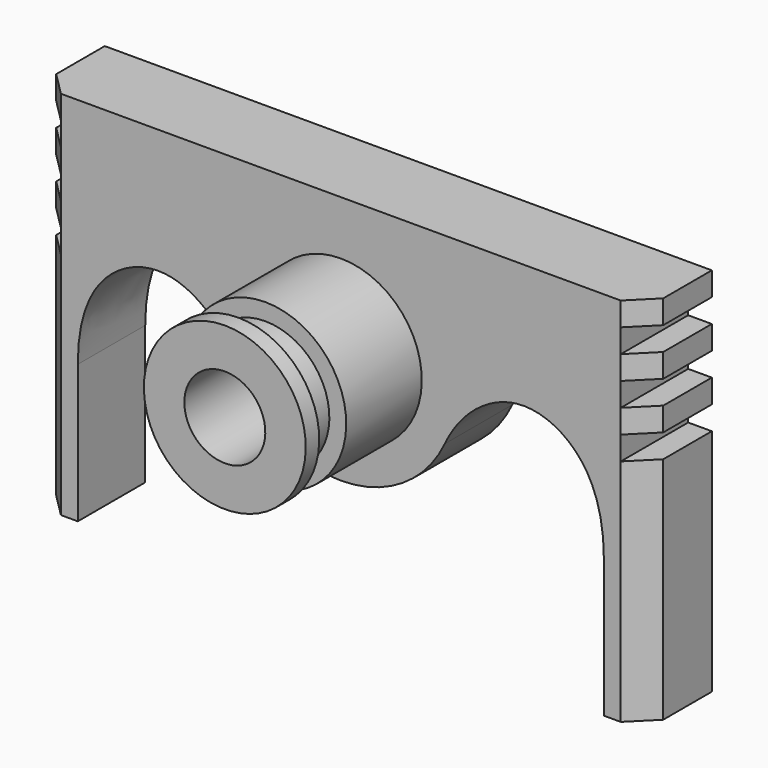
from build123d import *
from build123d import SkipClean  # not in build123d's __all__

# Parameters (mm, degrees)
F1_DEPTH = 2.5
F4_SIZE  = 0.7
F3_W     = 2.5
F3_H     = 1.2


with BuildPart() as f1:
    # F0 (on Front) → F1 (new body)
    with BuildSketch(Plane.XZ):
        with BuildLine():
            Line((0, 4), (-9, 4))
            Line((-9, 4), (-9, 3.3))
            Line((-9, 3.3), (-8.3, 3.3))
            Line((-8.3, 3.3), (-8.3, 2.6))
            Line((-8.3, 2.6), (-9, 2.6))
            Line((-9, 2.6), (-9, 1.9))
            Line((-9, 1.9), (-8.3, 1.9))
            Line((-8.3, 1.9), (-8.3, 1.2))
            Line((-8.3, 1.2), (-9, 1.2))
            Line((-9, 1.2), (-9, 0.5))
            Line((-9, 0.5), (-8.3, 0.5))
            Line((-8.3, 0.5), (-8.3, -0.2))
            Line((-8.3, -0.2), (-9, -0.2))
            Line((-9, -0.2), (-9, -7))
            Line((-9, -7), (-7.8, -7))
            Line((-7.8, -7), (-7.8, -2.900873477))
            add(Edge.make_bspline(
                [(-7.8, -2.900873477), (-7.8, -1.685574969), (-7.1826716424, -0.1281665724), (-4.9759016066, 0.6847768295), (-3.5267368498, -0.4819738014), (-3.0814464759, -1.4369020899)],
                knots=[0, 0, 0, 0, 0.3572792207, 0.6508868549, 1, 1, 1, 1], degree=3))
            ThreePointArc((-3.0814464759, -1.4369020899), (-1.8268186684, -2.8675309158), (0, -3.4))
            Line((0, -3.4), (0, -2.4))
            ThreePointArc((0, -2.4), (-2.4, 0), (0, 2.4))
            Line((0, 2.4), (0, 4))
        make_face()
    extrude(amount=F1_DEPTH)

    # F2: F1 across plane


with BuildPart() as f1_1:
    add(f1.part, clean=False)
    with SkipClean():  # cleaning this boolean's faces spoils the solid; the shape is the same uncleaned
        add(f1.part.mirror(Plane.YZ), clean=False)

    # F4
    f4_edges = [f1_1.edges().sort_by_distance(p)[0] for p in [
        (-9, -2.5, -3.6),
        (9, -2.5, -3.6),
        (-9, -2.5, 3.65),
        (-9, -2.5, 2.25),
        (-9, -2.5, 0.85),
        (9, -2.5, 3.65),
        (9, -2.5, 2.25),
        (9, -2.5, 0.85),
    ]]
    chamfer(f4_edges, length=F4_SIZE)

    # F3 (on Right) → F5 (revolve)
    with BuildSketch(Plane.YZ):
        Polygon((-2.5, 1.2), (-2.5, 2.4), (-5.3, 2.4), (-5.3, 1.9), (-6.3, 1.9), (-6.3, 2.4), (-6.8, 2.4), (-6.8, 1.2), align=None)
        with Locations((-1.25, 1.8)):
            Rectangle(F3_W, F3_H)
    revolve(axis=Axis((0, -3.9747959284, 0), (0, -1, 0)))


solid = f1_1.part
